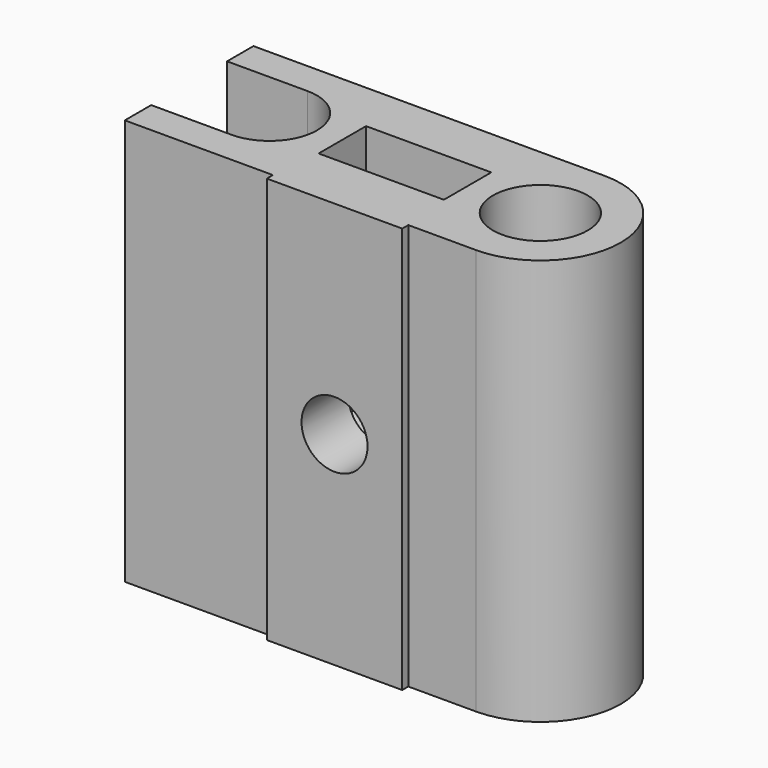
from build123d import *

# Parameters (mm, degrees)
F0_R     = 2.8
F0_W     = 8
F0_H     = 0.45
F1_DEPTH = 24
F2_R     = 1.95
F3_DEPTH = 9.951
F4_W     = 7.4
F4_H     = 3.5
F5_DEPTH = 12
F7_DEPTH = 3.5


# Not quite as in the source:
# - a feature names something its author has since deleted; it is built from what else it names


with BuildPart() as f1:
    # F0 (on Top) → F1 (new body)
    with BuildSketch(Plane.XY):
        with BuildLine():
            ThreePointArc((-8, 2.8), (-5.2, 0), (-8, -2.8))
            Line((-8, -2.8), (-12.75, -2.8))
            Line((-12.75, -2.8), (-12.75, -4.75))
            Line((-12.75, -4.75), (-8, -4.75))
            Line((-8, -4.75), (-4, -4.75))
            Line((-4, -4.75), (-4, -4.3))
            Line((-4, -4.3), (4, -4.3))
            Line((4, -4.3), (4, -4.75))
            Line((4, -4.75), (8, -4.75))
            ThreePointArc((8, -4.75), (12.75, 0), (8, 4.75))
            Line((8, 4.75), (-8, 4.75))
            Line((-8, 4.75), (-12.75, 4.75))
            Line((-12.75, 4.75), (-12.75, 2.8))
            Line((-12.75, 2.8), (-8, 2.8))
        make_face()
        with Locations((8, 0)):
            Circle(F0_R, mode=Mode.SUBTRACT)
        with Locations((0, -4.525)):
            Rectangle(F0_W, F0_H)
        with Locations((0, -4.975)):
            Rectangle(F0_W, F0_H)
    extrude(amount=F1_DEPTH)

    # F2 (on face) → F3 (cut, through all)
    with BuildSketch(Plane.XZ.offset(5.2)):
        with Locations((0, 12)):
            Circle(F2_R)
    extrude(amount=-F3_DEPTH, mode=Mode.SUBTRACT)

    # F4 (on face) → F5 (cut)
    with BuildSketch(Plane.XY.offset(24)):
        Rectangle(F4_W, F4_H)
    extrude(amount=-F5_DEPTH, mode=Mode.SUBTRACT)

    # F6 (on face) → F7 (cut, through all)
    with BuildSketch(Plane.XZ.offset(-1.75)):
        Polygon((3.7, 9.563804004), (3.7, 13.836195996), (0, 15.972391992), (-3.7, 13.836195996), (-3.7, 9.563804004), (0, 7.427608008), align=None)
    extrude(amount=F7_DEPTH, mode=Mode.SUBTRACT)


solid = f1.part
